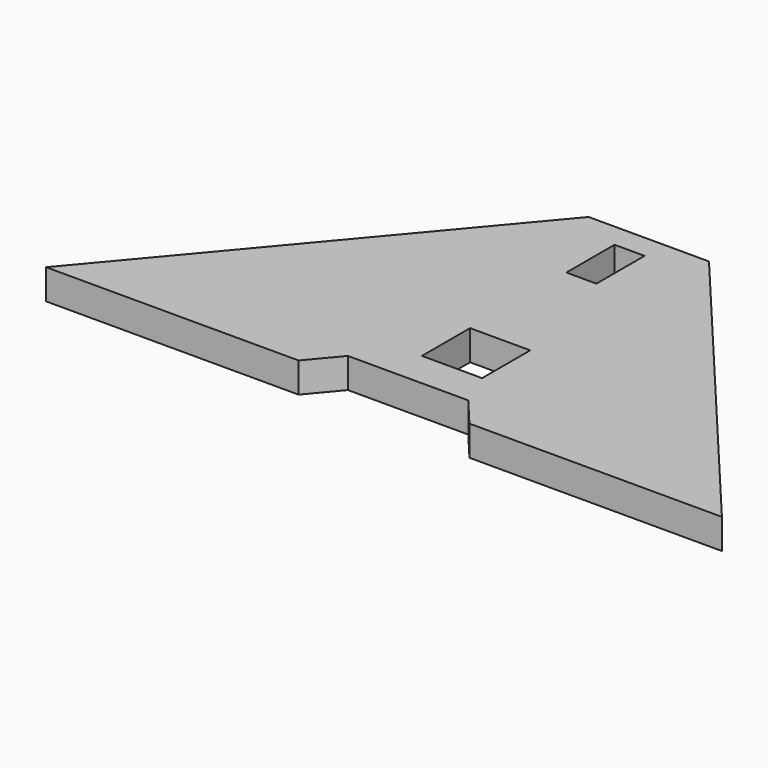
from build123d import *

# Parameters (mm, degrees)
F0_W     = 3.175
F0_H     = 6.35
F1_DEPTH = 3.175


# Not quite as in the source:
# - a length typed as a fraction of an inch, garbled in the dataset ("3 / 203.2 mm" for 3/8 in), is restored


with BuildPart() as f1:
    # F0 (on Top) → F1 (new body)
    with BuildSketch(Plane.XY):
        Polygon((6.35, 0), (-6.35, 0), (-35.6555546189, -34.925), (-9.014141329, -34.925), (-6.35, -31.75), (6.35, -31.75), (9.014141329, -34.925), (35.6555546189, -34.925), align=None)
        Polygon((-1.5875, -27.94), (-1.5875, -21.59), (1.5875, -21.59), (4.7625, -21.59), (4.7625, -27.94), (1.5875, -27.94), align=None, mode=Mode.SUBTRACT)
        with Locations((0, -5.715)):
            Rectangle(F0_W, F0_H, mode=Mode.SUBTRACT)
    extrude(amount=F1_DEPTH)


solid = f1.part
